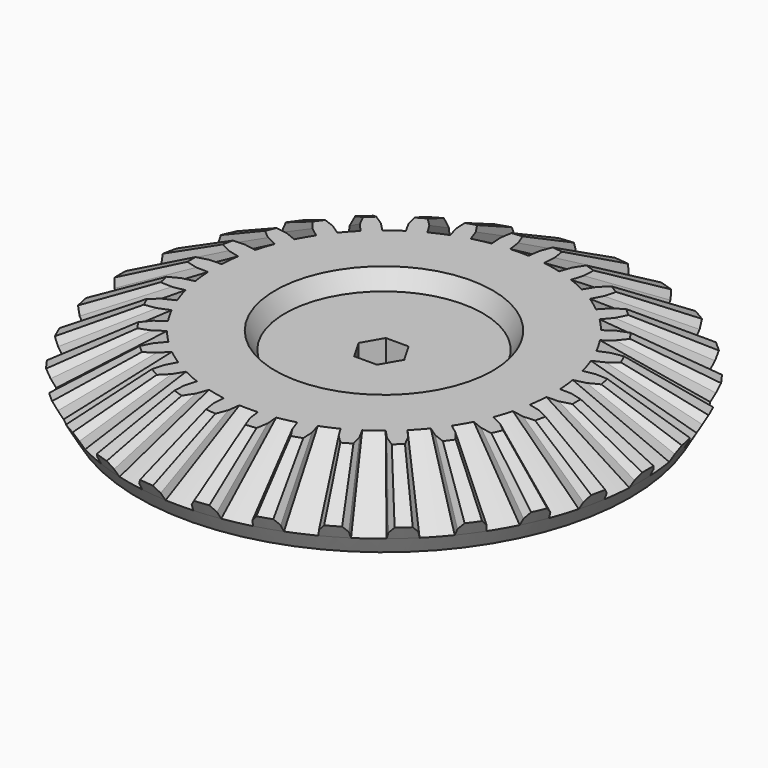
from build123d import *

# Parameters (mm, degrees)
F4_COPIES_COUNT = 30
F8_DEPTH        = 7.5977987664


# Not quite as in the source:
# - a pattern or mirror of a feature is missing from the dataset's text; its kind, count and spacing are read off the source's solid


with BuildPart() as f1:
    # F0 (on Front) → F1 (revolve)
    with BuildSketch(Plane.XZ):
        Polygon((0, 24.9992666559), (0, 0), (37.3, 0), (38.8, 2.5980762114), align=None)
    revolve(axis=Axis((0, 0, 12.499633328), (0, 0, -1)))

    # F3 (on line) → F4 section 0
    with BuildSketch(Plane(origin=(27.975, 0, -16.1513737806), x_dir=(0, -1, 0), z_dir=(-0.8660254038, 0, 0.5)), mode=Mode.PRIVATE) as f4_s0:
        with BuildLine():
            Line((-1.075, 24.05), (-1.7848764097, 22.9354417079))
            Line((-1.7848764097, 22.9354417079), (-1.9572102396, 21.6253021143))
            add(Edge.make_bspline(
                [(1.9572102396, 21.6253021143), (0, 21.6747293684), (-1.9572102396, 21.6253021143)],
                knots=[1.5203313467, 1.5203313467, 1.5203313467, 1.6212613069, 1.6212613069, 1.6212613069], degree=2, weights=[1, 0.9987269131, 1]))
            Line((1.9572102396, 21.6253021143), (1.7848764097, 22.9354417079))
            Line((1.7848764097, 22.9354417079), (1.075, 24.05))
            Line((1.075, 24.05), (0, 24.05))
            Line((0, 24.05), (-1.075, 24.05))
        make_face()
    f4 = loft([Vertex(0, 0, 24.9992666559), f4_s0.sketch])

    # F4_copies: F4 ×30 about axis
    f4_copies_axis = Axis((0, 0, 0), (0, 0, 1))
    for i in range(1, F4_COPIES_COUNT):
        add(f4.rotate(f4_copies_axis, i * 360 / F4_COPIES_COUNT))

    # F5 (on Front) → F6 (revolve, cut)
    with BuildSketch(Plane.XZ):
        Polygon((15, 7.5967987664), (16.4874144763, 10.1730762114), (35.9965173271, 10.1730762114), (41.4426787011, 7.1753299898), (37.3, 0), (44.386100024, 2.5980762114), (44.386100024, 8.9668417349), (0, 34.0423993766), (0, 7.5967987664), align=None)
    revolve(axis=Axis((0, 0, 20.8195990715), (0, 0, 1)), mode=Mode.SUBTRACT)

    # F7 (on face) → F8 (cut, through all)
    with BuildSketch(Plane.XY.offset(7.5967987664)):
        Polygon((1.7320508076, 2.5038056758), (-1.7320508076, 2.5038056758), (-3.4641016151, -0.4961943242), (-1.7320508076, -3.4961943242), (1.7320508076, -3.4961943242), (3.4641016151, -0.4961943242), align=None)
    extrude(amount=-F8_DEPTH, mode=Mode.SUBTRACT)


solid = f1.part
